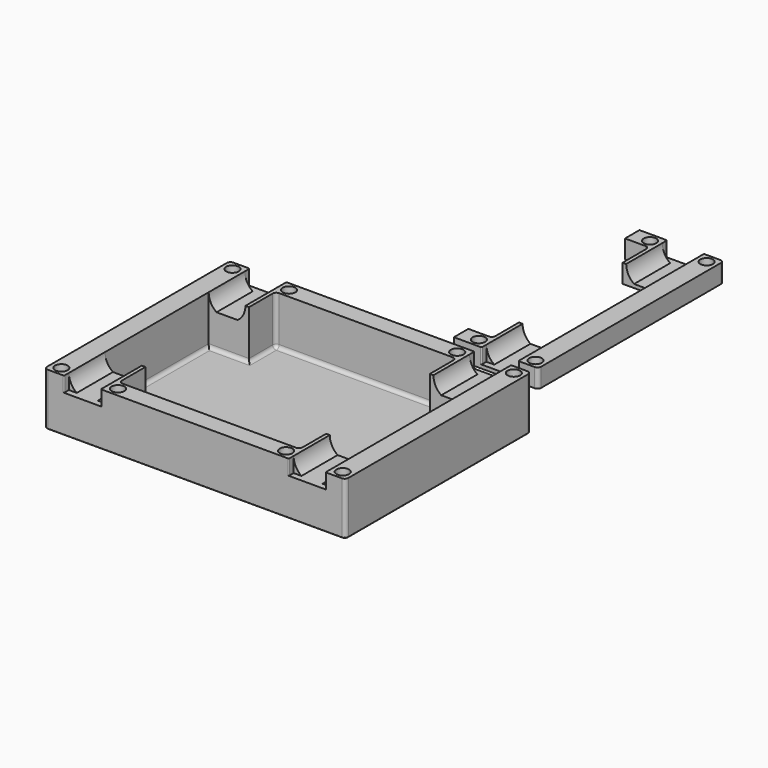
from build123d import *

# Parameters (mm, degrees)
F0_W         = 30
F0_H         = 32.5
F0_W_2       = 12.2
F0_H_2       = 21.5
F0_R         = 2.1
F0_H_3       = 15
F0_H_4       = 2
F1_DEPTH     = 12.4
F2_DEPTH     = 11.2
F3_DEPTH     = 5
F5_DEPTH     = 1.2
F7_DEPTH     = 15
F8_T1_DEPTH  = 24.5
F8_T3_DEPTH  = 15.2
F8_T5_DEPTH  = 10
F8_T7_DEPTH  = 5
F8_T9_DEPTH  = 9.8
F8_T11_DEPTH = 28.8
F8_T13_DEPTH = 1.2
F8_S17_W     = 1.2
F8_S17_H     = 1.2
F8_T18_DEPTH = 1.2
F8_T25_DEPTH = 4.2
F8_T29_DEPTH = 12.8
F8_T32_DEPTH = 23.4
F9_R         = 0.3
F14_DEPTH    = 77


# Not quite as in the source:
# - a fillet or chamfer that OpenCascade refuses, or shapes differently, is made with other operations: its cross-section is extruded or revolved along the edge and cut away or added


with BuildPart() as f1:
    # F0 (on Top) → F1 (new body)
    with BuildSketch(Plane.XY):
        Polygon((-30, 32.5), (0, 32.5), (0, 38.5), (-30, 38.5), (-30, 35.5), align=None)
        with BuildLine():
            ThreePointArc((-25.8, 35.5), (-27.9, 33.4), (-30, 35.5))
            ThreePointArc((-30, 35.5), (-27.9, 37.6), (-25.8, 35.5))
        make_face(mode=Mode.SUBTRACT)
        with Locations((-15, 16.25)):
            Rectangle(F0_W, F0_H)
        with Locations((-37.3, 10.75)):
            Rectangle(F0_W_2, F0_H_2)
        Polygon((-50, 0), (-43.4, 0), (-43.4, 21.5), (-43.4, 36.5), (-43.4, 38.5), (-50, 38.5), align=None)
        with Locations((-46.7, 35.5)):
            Circle(F0_R, mode=Mode.SUBTRACT)
        with Locations((-37.3, 29)):
            Rectangle(F0_W_2, F0_H_3)
        with Locations((-37.3, 37.5)):
            Rectangle(F0_W_2, F0_H_4)
        Polygon((-31.2, 0), (-30, 0), (-30, 32.5), (-30, 35.5), (-30, 38.5), (-31.2, 38.5), (-31.2, 36.5), (-31.2, 21.5), align=None)
    extrude(amount=-F1_DEPTH)

    # F0 (on Top) → F2 (cut)
    with BuildSketch(Plane.XY):
        with Locations((-15, 16.25)):
            Rectangle(F0_W, F0_H)
        with Locations((-37.3, 10.75)):
            Rectangle(F0_W_2, F0_H_2)
    extrude(amount=-F2_DEPTH, mode=Mode.SUBTRACT)

    # F0 (on Top) → F3 (join)
    with BuildSketch(Plane.XY):
        Polygon((-30, 32.5), (0, 32.5), (0, 38.5), (-30, 38.5), (-30, 35.5), align=None)
        with BuildLine():
            ThreePointArc((-25.8, 35.5), (-27.9, 33.4), (-30, 35.5))
            ThreePointArc((-30, 35.5), (-27.9, 37.6), (-25.8, 35.5))
        make_face(mode=Mode.SUBTRACT)
        Polygon((-31.2, 0), (-30, 0), (-30, 32.5), (-30, 35.5), (-30, 38.5), (-31.2, 38.5), (-31.2, 36.5), (-31.2, 21.5), align=None)
        Polygon((-50, 0), (-43.4, 0), (-43.4, 21.5), (-43.4, 36.5), (-43.4, 38.5), (-50, 38.5), align=None)
        with Locations((-46.7, 35.5)):
            Circle(F0_R, mode=Mode.SUBTRACT)
    extrude(amount=F3_DEPTH)

    # F4 (on face) → F5 (cut, through all)
    with BuildSketch(Plane(origin=(-31.2, 0, 0), x_dir=(0, -1, 0), z_dir=(-1, 0, 0))):
        Polygon((-21.5, 0), (-21.5, -11.2), (0, -11.2), (0, 5), (-21.5, 5), align=None)
    extrude(amount=-F5_DEPTH, mode=Mode.SUBTRACT)

    # F6 (on face) → F7 (join)
    with BuildSketch(Plane.XZ.offset(-21.5)):
        with BuildLine():
            ThreePointArc((-31.2, 5), (-31.8905122999, 2.1808790693), (-33.8057189581, 0))
            Line((-33.8057189581, 0), (-31.2, 0))
            Line((-31.2, 0), (-31.2, 5))
        make_face()
        with BuildLine():
            ThreePointArc((-40.7942810419, 0), (-42.7094877001, 2.1808790693), (-43.4, 5))
            Line((-43.4, 5), (-43.4, 0))
            Line((-43.4, 0), (-40.7942810419, 0))
        make_face()
    extrude(amount=-F7_DEPTH)

    # F8: fillet of radius 1.2 on 9 edges, made by hand

    # F8_s2 → F8_t1 (join)
    with BuildSketch(Plane.XZ.offset(-24.5)):
        with BuildLine():
            ThreePointArc((-43.4, -10), (-43.0485281374, -10.8485281374), (-42.2, -11.2))
            Line((-42.2, -11.2), (-43.4, -11.2))
            Line((-43.4, -11.2), (-43.4, -10))
        make_face()
    extrude(amount=F8_T1_DEPTH)

    # F8_s4 → F8_t3 (join)
    with BuildSketch(Plane.YZ.offset(-46.4)):
        with BuildLine():
            ThreePointArc((21.5, -10), (21.1485281374, -10.8485281374), (20.3, -11.2))
            Line((20.3, -11.2), (21.5, -11.2))
            Line((21.5, -11.2), (21.5, -10))
        make_face()
    extrude(amount=F8_T3_DEPTH)

    # F8_s6 → F8_t5 (join)
    with BuildSketch(Plane.XY.offset(-10)):
        with BuildLine():
            ThreePointArc((-28.8, 32.5), (-29.6485281374, 32.1485281374), (-30, 31.3))
            Line((-30, 31.3), (-30, 32.5))
            Line((-30, 32.5), (-28.8, 32.5))
        make_face()
    extrude(amount=F8_T5_DEPTH)

    # F8_s8 → F8_t7 (join)
    with BuildSketch(Plane.XY):
        with BuildLine():
            ThreePointArc((-28.8, 32.5), (-29.6485281374, 32.1485281374), (-30, 31.3))
            Line((-30, 31.3), (-30, 32.5))
            Line((-30, 32.5), (-28.8, 32.5))
        make_face()
    extrude(amount=F8_T7_DEPTH)

    # F8_s10 → F8_t9 (join)
    with BuildSketch(Plane.XZ.offset(-31.3)):
        with BuildLine():
            ThreePointArc((-28.8, -11.2), (-29.6485281374, -10.8485281374), (-30, -10))
            Line((-30, -10), (-30, -11.2))
            Line((-30, -11.2), (-28.8, -11.2))
        make_face()
    extrude(amount=F8_T9_DEPTH)

    # F8_s12 → F8_t11 (join)
    with BuildSketch(Plane.YZ.offset(-28.8)):
        with BuildLine():
            ThreePointArc((32.5, -10), (32.1485281374, -10.8485281374), (31.3, -11.2))
            Line((31.3, -11.2), (32.5, -11.2))
            Line((32.5, -11.2), (32.5, -10))
        make_face()
    extrude(amount=F8_T11_DEPTH)

    # F8_s14 → F8_t13 (join)
    with BuildSketch(Plane.YZ.offset(-31.2)):
        with BuildLine():
            ThreePointArc((21.5, -10), (21.1485281374, -10.8485281374), (20.3, -11.2))
            Line((20.3, -11.2), (21.5, -11.2))
            Line((21.5, -11.2), (21.5, -10))
        make_face()
    extrude(amount=F8_T13_DEPTH)


with BuildPart() as f8_tool16:
    # F8_s17 → F8_t18 (new body)
    with BuildSketch(Plane.YZ.offset(-28.8)):
        with Locations((31.9, -10.6)):
            Rectangle(F8_S17_W, F8_S17_H)
    extrude(amount=-F8_T18_DEPTH)

    # F8_s19 → F8_t20 (revolve, cut)
    with BuildSketch(Plane(origin=(-28.8, 31.3, -10), x_dir=(0, -0.7071067812, 0.7071067812), z_dir=(0, -0.7071067812, -0.7071067812))):
        with BuildLine():
            ThreePointArc((0, -1.2), (1.2, 0), (0, 1.2))
            Line((0, 1.2), (0, -1.2))
        make_face()
    revolve(axis=Axis((-28.8, 31.3, -10), (-1, 0, 0)), mode=Mode.SUBTRACT)


with BuildPart() as f1_1:
    add(f1.part)

    # F8_t15: union F8_tool16
    add(f8_tool16.part)


with BuildPart() as f8_tool23:
    # F8_s24 → F8_t25 (new body)
    with BuildSketch(Plane.YZ.offset(-31.2)):
        with BuildLine():
            ThreePointArc((21.5, -10), (21.1485281374, -10.8485281374), (20.3, -11.2))
            Line((20.3, -11.2), (21.5, -11.2))
            Line((21.5, -11.2), (21.5, -10))
        make_face()
    extrude(amount=F8_T25_DEPTH)

    split(bisect_by=Plane.YZ.offset(-30), keep=Keep.TOP)


with BuildPart() as f8_tool27:
    # F8_s28 → F8_t29 (new body)
    with BuildSketch(Plane.XZ.offset(-31.3)):
        with BuildLine():
            ThreePointArc((-28.8, -11.2), (-29.6485281374, -10.8485281374), (-30, -10))
            Line((-30, -10), (-30, -11.2))
            Line((-30, -11.2), (-28.8, -11.2))
        make_face()
    extrude(amount=F8_T29_DEPTH)

    split(bisect_by=Plane.XZ.offset(-21.5), keep=Keep.TOP)


with BuildPart() as f8_tool23_1:
    add(f8_tool23.part)

    # F8_t31: intersect F8_tool27
    add(f8_tool27.part, mode=Mode.INTERSECT)


with BuildPart() as f1_2:
    add(f1_1.part)

    # F8_t21: union F8_tool23
    add(f8_tool23_1.part)

    # F8_s33 → F8_t32 (cut)
    with BuildSketch(Plane.XY.offset(-15.4)):
        with BuildLine():
            ThreePointArc((-48.8, 38.5), (-49.6485281374, 38.1485281374), (-50, 37.3))
            Line((-50, 37.3), (-50, 38.5))
            Line((-50, 38.5), (-48.8, 38.5))
        make_face()
    extrude(amount=F8_T32_DEPTH, mode=Mode.SUBTRACT)

    # F9
    f9_edges = [f1_2.edges().sort_by_distance(p)[0] for p in [
        (-50, 18.65, -12.4),
        (-31.2, 38.5, 2.5),
        (-43.4, 38.5, 2.5),
        (-24.4, 38.5, -12.4),
        (-49.648528, 38.148528, -12.4),
    ]]
    fillet(f9_edges, radius=F9_R)

    # F10: F1 across face


with BuildPart() as f1_3:
    add(f1_2.part)
    add(f1_2.part.mirror(Plane(origin=(-38.9064033059, 0, -6.2352362766), x_dir=(1, 0, 0), z_dir=(0, -1, 0))))

    # F11: F1 across face


with BuildPart() as f1_4:
    add(f1_3.part)
    add(f1_3.part.mirror(Plane(origin=(0, 0, -5.9128802639), x_dir=(0, 1, 0), z_dir=(1, 0, 0))))


with BuildPart() as f12_1:
    # F12: copy of F1
    add(f1_4.part.moved(Location((0, 80, 0))))

    # F13 (on face) → F14 (cut, through all)
    with BuildSketch(Plane.XZ.offset(-41.5)):
        Polygon((50, -12.1), (50, -1.2), (22, -1.2), (22, -12.4), (48.8, -12.4), (50, -12.4), align=None)
        Polygon((22, -12.4), (22, -1.2), (22, 5), (-50, 5), (-50, -12.1), (-50, -12.4), (-48.8, -12.4), align=None)
    extrude(amount=-F14_DEPTH, mode=Mode.SUBTRACT)


solid = Compound([f1_4.part, f12_1.part])
